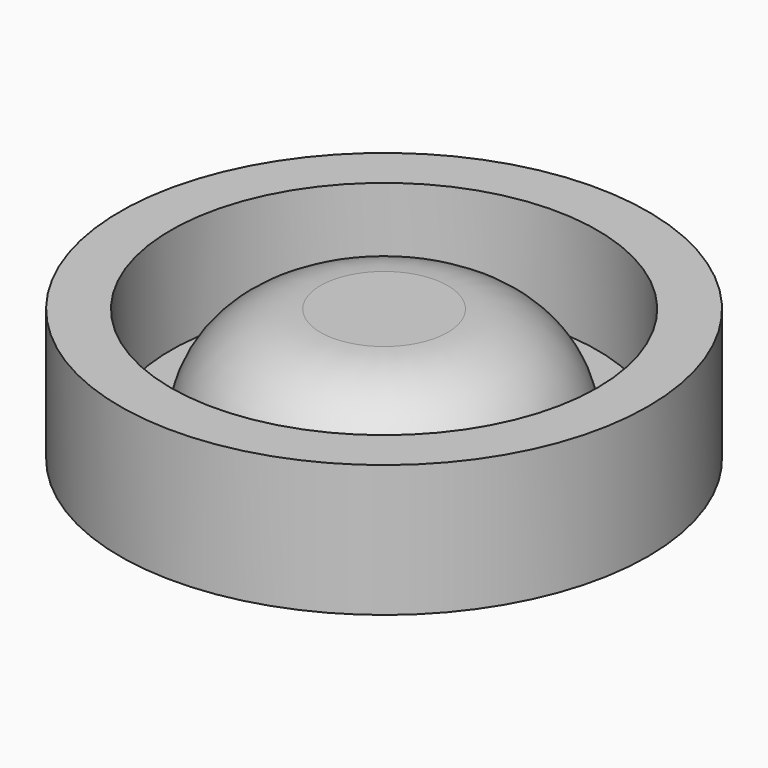
from build123d import *

# Parameters (mm, degrees)
F0_R     = 25.4
F1_DEPTH = 12.7
F2_R     = 20.5279895556
F3_DEPTH = 10.16
F4_R     = 16.2758477469
F5_DEPTH = 10.16
F6_R     = 10.15999


# Not quite as in the source:
# - a fillet or chamfer is up to 0.001 mm smaller than in the source, because OpenCascade refuses the exact size


with BuildPart() as f1:
    # F0 (on Top) → F1 (new body)
    with BuildSketch(Plane.XY):
        Circle(F0_R)
    extrude(amount=F1_DEPTH)

    # F2 (on face) → F3 (cut)
    with BuildSketch(Plane.XY.offset(12.7)):
        Circle(F2_R)
    extrude(amount=-F3_DEPTH, mode=Mode.SUBTRACT)

    # F4 (on face) → F5 (join)
    with BuildSketch(Plane.XY.offset(2.54)):
        Circle(F4_R)
    extrude(amount=F5_DEPTH)

    # F6 (radius 10.16 in the source; OpenCascade refuses exactly that, so slightly less here)
    f6_edges = [f1.edges().sort_by_distance(p)[0] for p in [
        (-16.275848, 0, 12.7),
    ]]
    fillet(f6_edges, radius=F6_R)


solid = f1.part
